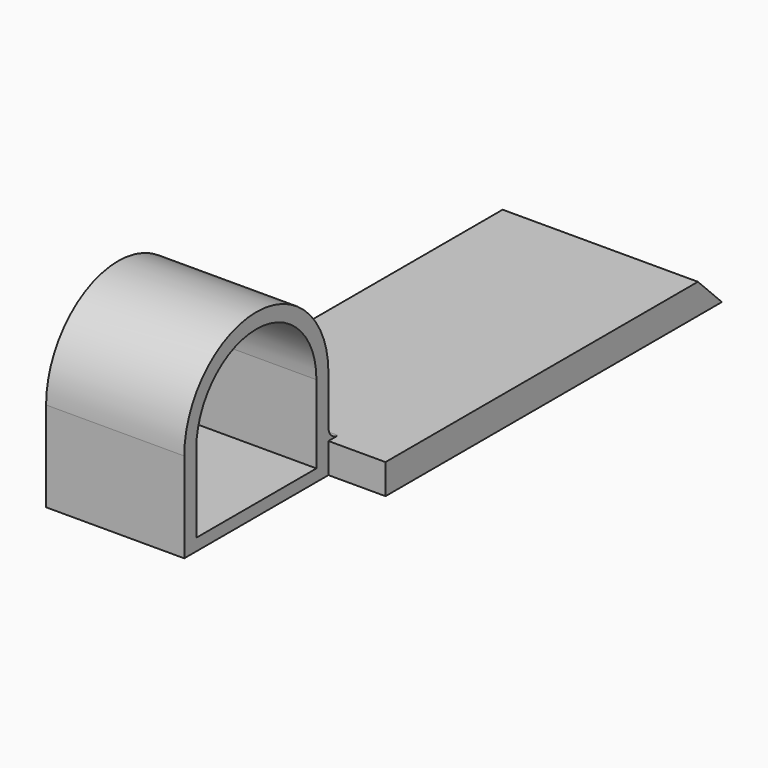
from build123d import *

# Parameters (mm, degrees)
F1_W      = 0.5
F1_H      = 7.5
F1_H_2    = 1
F2_DEPTH  = 11
F1_W_2    = 25
F1_H_3    = 2
F3_DEPTH  = 2.5
F6_DEPTH  = 1
F1_W_3    = 70
F1_H_4    = 5
F7_DEPTH  = 23
F9_W      = 70
F9_H      = 5
F10_DEPTH = 12.5
F11_SIZE  = 4.99999
F13_R     = 2


# Not quite as in the source:
# - a fillet or chamfer is up to 0.001 mm smaller than in the source, because OpenCascade refuses the exact size


with BuildPart() as f2:
    # F1 (on offset) → F2 (new body)
    with BuildSketch(Plane.YZ.offset(-27.5)):
        Polygon((-26, 6), (-26, 15), (-27, 15), (-27, 5), (-22, 5), (-22, 7.5), (-22.5, 7.5), (-22.5, 15), (-23, 15), (-23, 6), align=None)
        Polygon((-27, 15), (-26, 15), (-23, 15), (-22.5, 15), (-22.5, 16), (-27, 16), align=None)
        with Locations((-22.25, 11.25)):
            Rectangle(F1_W, F1_H)
        with Locations((-22.25, 15.5)):
            Rectangle(F1_W, F1_H_2)
    extrude(amount=F2_DEPTH)

    # F1 (on offset) → F3 (join)
    with BuildSketch(Plane.YZ.offset(-27.5)):
        with BuildLine():
            Line((-27.5, 2), (-2.5, 2))
            Line((-2.5, 2), (-2.5, 15))
            ThreePointArc((-2.5, 15), (-15, 27.5), (-27.5, 15))
            Line((-27.5, 15), (-27.5, 2))
        make_face()
        Polygon((-27, 5), (-27, 15), (-27, 16), (-22.5, 16), (-22.5, 22.5), (-7.5, 22.5), (-7.5, 7.5), (-22, 7.5), (-22, 5), align=None, mode=Mode.SUBTRACT)
        Polygon((-22, 16), (-22, 15), (-22, 7.5), (-7.5, 7.5), (-7.5, 22.5), (-22.5, 22.5), (-22.5, 16), align=None)
        with Locations((-15, 1)):
            Rectangle(F1_W_2, F1_H_3)
    extrude(amount=F3_DEPTH)

    # F5 (on offset) → F6 (join)
    with BuildSketch(Plane.YZ.offset(-16.5)):
        Polygon((-26, 14), (-26, 15), (-23, 15), (-23, 13.8), (-22, 16), (-27, 16), (-27, 5), (-26, 7.2), align=None)
        Polygon((-26, 6), (-26, 7.2), (-27, 5), (-25, 5), (-24, 5), (-22, 5), (-22, 16), (-23, 13.8), (-23, 6), align=None)
        Polygon((-23, 15), (-26, 15), (-26, 14), (-26, 7.2), (-25, 9.4), (-25, 14.75), (-24, 14.75), (-24, 11.6), (-23, 13.8), align=None)
        Polygon((-25, 9.4), (-26, 7.2), (-26, 6), (-23, 6), (-23, 13.8), (-24, 11.6), (-24, 6.25), (-25, 6.25), align=None)
    extrude(amount=F6_DEPTH)

    # F1 (on offset) → F7 (join)
    with BuildSketch(Plane.YZ.offset(-27.5)):
        with BuildLine():
            Line((-2.5, 0), (0, 0))
            Line((0, 0), (0, 5))
            Line((0, 5), (0, 15))
            ThreePointArc((0, 15), (-15, 30), (-30, 15))
            Line((-30, 15), (-30, 0))
            Line((-30, 0), (-27.5, 0))
            Line((-27.5, 0), (-27.5, 2))
            Line((-27.5, 2), (-27.5, 15))
            ThreePointArc((-27.5, 15), (-15, 27.5), (-2.5, 15))
            Line((-2.5, 15), (-2.5, 2))
            Line((-2.5, 2), (-2.5, 0))
        make_face()
        with Locations((35, 2.5)):
            Rectangle(F1_W_3, F1_H_4)
        with Locations((-15, 1)):
            Rectangle(F1_W_2, F1_H_3)
    extrude(amount=F7_DEPTH)

    # F9 (on offset) → F10 (join)
    with BuildSketch(Plane.YZ.offset(-7.5)):
        with Locations((35, 2.5)):
            Rectangle(F9_W, F9_H)
    extrude(amount=F10_DEPTH)

    # F11 (size 5 in the source; OpenCascade refuses exactly that, so slightly less here)
    f11_edges = [f2.edges().sort_by_distance(p)[0] for p in [
        (-11.25, 70, 5),
    ]]
    chamfer(f11_edges, length=F11_SIZE)

    # F13
    f13_edges = [f2.edges().sort_by_distance(p)[0] for p in [
        (-16, 0, 5),
    ]]
    fillet(f13_edges, radius=F13_R)


solid = f2.part
